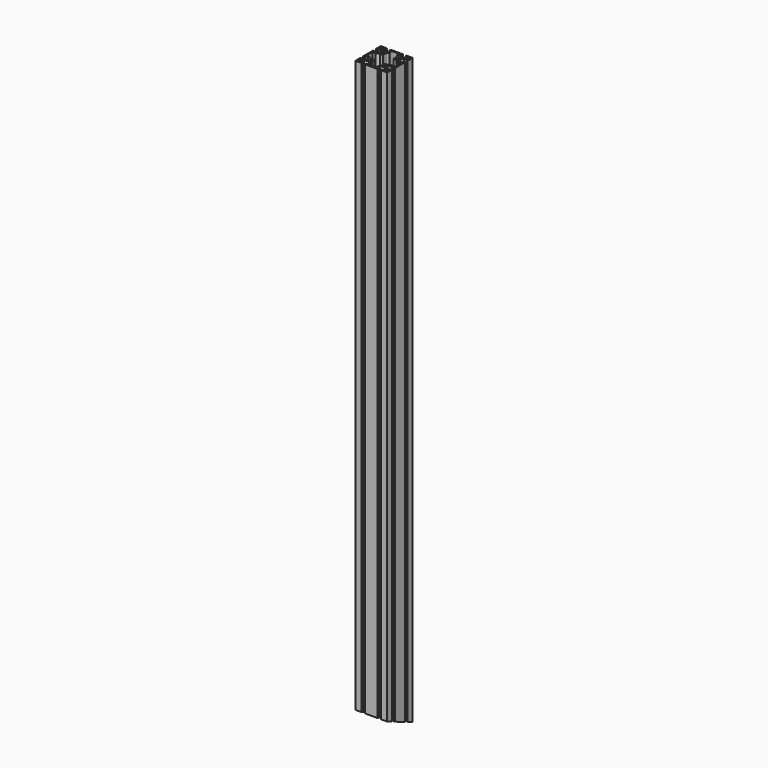
from build123d import *

# Parameters (mm, degrees)
F0_R          = 3
F0_R_2        = 2.5
F1_DEPTH      = 1100.6
F2_R          = 2
F3_R          = 7
F5_DEPTH      = 30
F5_DEPTH_BACK = 30


# Not quite as in the source:
# - a feature names something its author has since deleted; it is built from what else it names


with BuildPart() as f1:
    # F0 (on Top) → F1 (new body)
    with BuildSketch(Plane.XY):
        with BuildLine():
            Line((18.15, -30), (30, -30))
            Line((30, -30), (30, -18.15))
            Line((30, -18.15), (27.5, -18.15))
            Line((27.5, -18.15), (27.5, -20.15))
            Line((27.5, -20.15), (21.5477069044, -20.15))
            ThreePointArc((21.5477069044, -20.15), (19.5, -15), (21.5477069044, -9.85))
            Line((21.5477069044, -9.85), (27.5, -9.85))
            Line((27.5, -9.85), (27.5, -11.85))
            Line((27.5, -11.85), (30, -11.85))
            Line((30, -11.85), (30, 11.85))
            Line((30, 11.85), (27.5, 11.85))
            Line((27.5, 11.85), (27.5, 9.85))
            Line((27.5, 9.85), (21.5477069044, 9.85))
            ThreePointArc((21.5477069044, 9.85), (19.5, 15), (21.5477069044, 20.15))
            Line((21.5477069044, 20.15), (27.5, 20.15))
            Line((27.5, 20.15), (27.5, 18.15))
            Line((27.5, 18.15), (30, 18.15))
            Line((30, 18.15), (30, 30))
            Line((30, 30), (18.15, 30))
            Line((18.15, 30), (18.15, 27.5))
            Line((18.15, 27.5), (20.15, 27.5))
            Line((20.15, 27.5), (20.15, 21.5477069044))
            ThreePointArc((20.15, 21.5477069044), (15, 19.5), (9.85, 21.5477069044))
            Line((9.85, 21.5477069044), (9.85, 27.5))
            Line((9.85, 27.5), (11.85, 27.5))
            Line((11.85, 27.5), (11.85, 30))
            Line((11.85, 30), (-11.85, 30))
            Line((-11.85, 30), (-11.85, 27.5))
            Line((-11.85, 27.5), (-9.85, 27.5))
            Line((-9.85, 27.5), (-9.85, 21.5477069044))
            ThreePointArc((-9.85, 21.5477069044), (-15, 19.5), (-20.15, 21.5477069044))
            Line((-20.15, 21.5477069044), (-20.15, 27.5))
            Line((-20.15, 27.5), (-18.15, 27.5))
            Line((-18.15, 27.5), (-18.15, 30))
            Line((-18.15, 30), (-30, 30))
            Line((-30, 30), (-30, 18.15))
            Line((-30, 18.15), (-27.5, 18.15))
            Line((-27.5, 18.15), (-27.5, 20.15))
            Line((-27.5, 20.15), (-21.5477069044, 20.15))
            ThreePointArc((-21.5477069044, 20.15), (-19.5, 15), (-21.5477069044, 9.85))
            Line((-21.5477069044, 9.85), (-27.5, 9.85))
            Line((-27.5, 9.85), (-27.5, 11.85))
            Line((-27.5, 11.85), (-30, 11.85))
            Line((-30, 11.85), (-30, -11.85))
            Line((-30, -11.85), (-27.5, -11.85))
            Line((-27.5, -11.85), (-27.5, -9.85))
            Line((-27.5, -9.85), (-21.5477069044, -9.85))
            ThreePointArc((-21.5477069044, -9.85), (-19.5, -15), (-21.5477069044, -20.15))
            Line((-21.5477069044, -20.15), (-27.5, -20.15))
            Line((-27.5, -20.15), (-27.5, -18.15))
            Line((-27.5, -18.15), (-30, -18.15))
            Line((-30, -18.15), (-30, -30))
            Line((-30, -30), (-18.15, -30))
            Line((-18.15, -30), (-18.15, -27.5))
            Line((-18.15, -27.5), (-20.15, -27.5))
            Line((-20.15, -27.5), (-20.15, -21.5477069044))
            ThreePointArc((-20.15, -21.5477069044), (-15, -19.5), (-9.85, -21.5477069044))
            Line((-9.85, -21.5477069044), (-9.85, -27.5))
            Line((-9.85, -27.5), (-11.85, -27.5))
            Line((-11.85, -27.5), (-11.85, -30))
            Line((-11.85, -30), (11.85, -30))
            Line((11.85, -30), (11.85, -27.5))
            Line((11.85, -27.5), (9.85, -27.5))
            Line((9.85, -27.5), (9.85, -21.5477069044))
            ThreePointArc((9.85, -21.5477069044), (15, -19.5), (20.15, -21.5477069044))
            Line((20.15, -21.5477069044), (20.15, -27.5))
            Line((20.15, -27.5), (18.15, -27.5))
            Line((18.15, -27.5), (18.15, -30))
        make_face()
        with Locations((-25, -25)):
            Circle(F0_R, mode=Mode.SUBTRACT)
        with Locations((-15, -15)):
            Circle(F0_R_2, mode=Mode.SUBTRACT)
        with Locations((25, -25)):
            Circle(F0_R, mode=Mode.SUBTRACT)
        with Locations((15, -15)):
            Circle(F0_R_2, mode=Mode.SUBTRACT)
        with Locations((-25, 25)):
            Circle(F0_R, mode=Mode.SUBTRACT)
        with Locations((-15, 15)):
            Circle(F0_R_2, mode=Mode.SUBTRACT)
        Polygon((-7, 22), (-7, 27.5), (0, 27.5), (7, 27.5), (7, 22), (10, 16), (10, 10), (16, 10), (22, 7), (27.5, 7), (27.5, 0), (27.5, -7), (22, -7), (16, -10), (10, -10), (10, -16), (7, -22), (7, -27.5), (0, -27.5), (-7, -27.5), (-7, -22), (-10, -16), (-10, -10), (-16, -10), (-22, -7), (-27.5, -7), (-27.5, 0), (-27.5, 7), (-22, 7), (-16, 10), (-10, 10), (-10, 16), align=None, mode=Mode.SUBTRACT)
        with Locations((15, 15)):
            Circle(F0_R_2, mode=Mode.SUBTRACT)
        with Locations((25, 25)):
            Circle(F0_R, mode=Mode.SUBTRACT)
    extrude(amount=F1_DEPTH)

    # F2
    f2_edges = [f1.edges().sort_by_distance(p)[0] for p in [
        (-7, 27.5, 550.3),
        (7, 27.5, 550.3),
    ]]
    fillet(f2_edges, radius=F2_R)

    # F3
    f3_edges = [f1.edges().sort_by_distance(p)[0] for p in [
        (-10, 16, 550.3),
        (10, 16, 550.3),
    ]]
    fillet(f3_edges, radius=F3_R)

    # F4 (on Right) → F5 (cut, two sides)
    with BuildSketch(Plane.YZ) as f5_sk:
        Polygon((-153.0130330148, 75.8064803658), (-200.6900714338, -39.2960723993), (-17.6770384191, -115.1025527651), (30, 0), align=None)
    extrude(amount=F5_DEPTH, mode=Mode.SUBTRACT)
    extrude(f5_sk.sketch, amount=-F5_DEPTH_BACK, mode=Mode.SUBTRACT)


solid = f1.part
